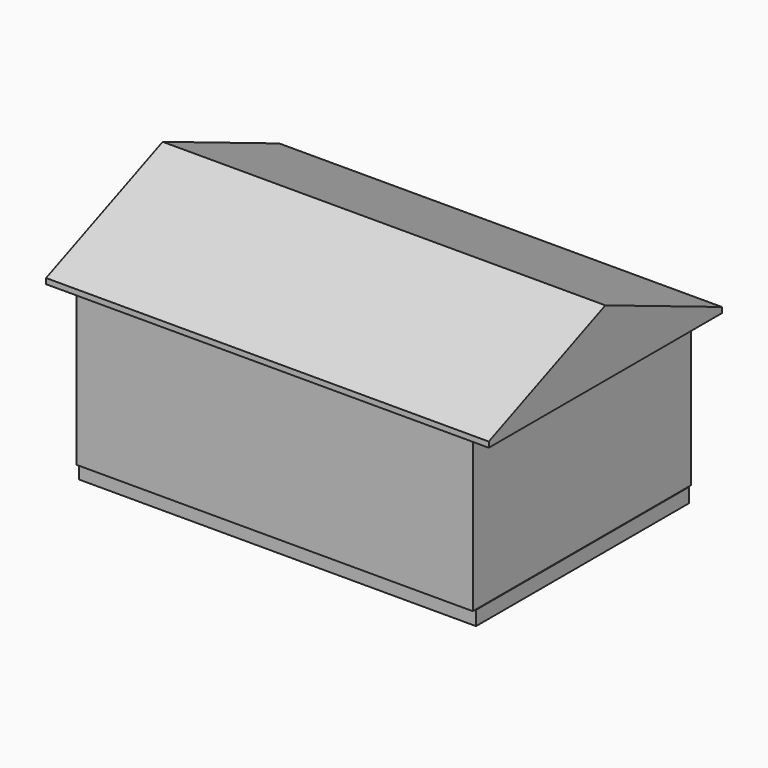
from build123d import *

# Parameters (mm, degrees)
F0_W        = 138.1315141916
F0_H        = 54.1731398553
F1_DEPTH    = 47.498
F0_H_2      = 6.7966300994
F2_DEPTH    = 50.8
F3_T1_DEPTH = 534.0028075166
F4_DEPTH    = 46.355


# Not quite as in the source:
# - a fillet or chamfer that OpenCascade refuses, or shapes differently, is made with other operations: its cross-section is extruded or revolved along the edge and cut away or added


with BuildPart() as f1:
    # F0 (on Front) → F1 (new body, symmetric)
    with BuildSketch(Plane.XZ):
        with Locations((0, -3.3983150497)):
            Rectangle(F0_W, F0_H)
    extrude(amount=F1_DEPTH, both=True)

    # F0 (on Front) → F4 (join, symmetric)
    with BuildSketch(Plane.XZ):
        Polygon((69.0657570958, -30.4848849773), (-69.0657570958, -30.4848849773), (-69.0657570958, -35.4824028909), (69.2656487226, -35.4824028909), (69.2656487226, -30.4848849773), align=None)
    extrude(amount=F4_DEPTH, both=True)


with BuildPart() as f2:
    # F0 (on Front) → F2 (new body, symmetric)
    with BuildSketch(Plane.XZ):
        with Locations((0, 27.0865699276)):
            Rectangle(F0_W, F0_H_2)
        Polygon((-69.0657570958, 23.6882548779), (-69.0657570958, 30.4848849773), (69.0657570958, 30.4848849773), (69.0657570958, 23.6882548779), (77.2616863251, 23.6882548779), (77.2616863251, 56.0721941292), (-77.0617872477, 56.0721941292), (-77.0617872477, 23.6882548779), align=None)
    extrude(amount=F2_DEPTH, both=True)

    # F3: chamfer of 30.48 x 73.2234970305 on 2 edges, made by hand

    # F3_s2 → F3_t1 (cut)
    with BuildSketch(Plane.YZ.offset(-266.9014542196)):
        Polygon((-22.4234970305, 56.0721941292), (50.8, 25.5921941292), (50.8, 56.0721941292), align=None)
        Polygon((-50.8, 25.5921941292), (22.4234970305, 56.0721941292), (-50.8, 56.0721941292), align=None)
    extrude(amount=F3_T1_DEPTH, mode=Mode.SUBTRACT)


solid = Compound([f1.part, f2.part])
